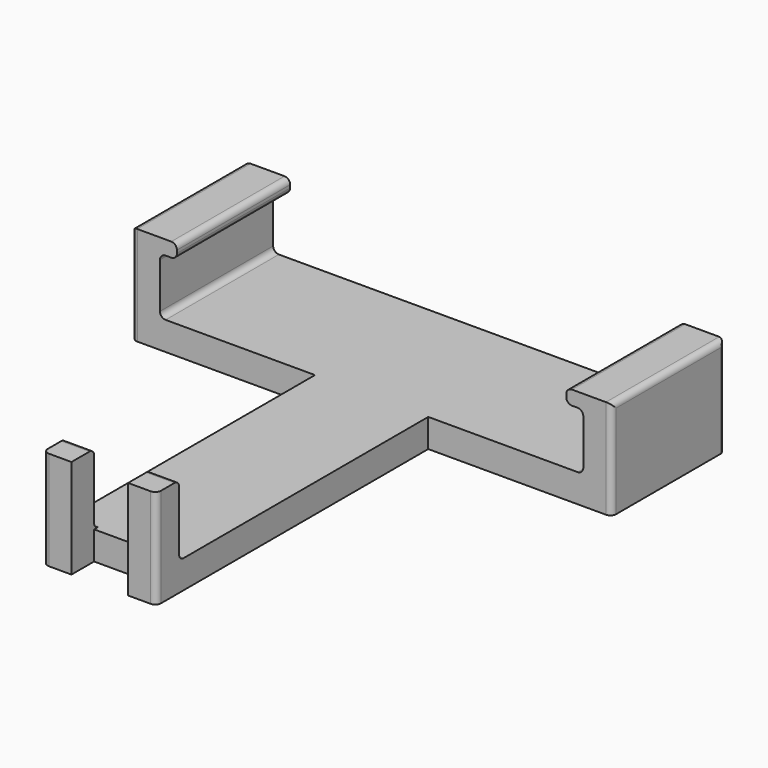
from build123d import *

# Parameters (mm, degrees)
F0_W     = 27.375
F0_H     = 25
F0_W_2   = 20
F0_H_2   = 55
F1_DEPTH = 5
F2_W     = 5
F2_H     = 25
F2_H_2   = 5
F3_DEPTH = 17.5
F4_W     = 25
F4_H     = 2.5
F5_DEPTH = 3
F6_W     = 25
F6_H     = 2.5
F7_DEPTH = 3
F8_R     = 1


with BuildPart() as f1:
    # F0 (on Top) → F1 (new body)
    with BuildSketch(Plane.XY):
        with Locations((-23.6875, 0)):
            Rectangle(F0_W, F0_H)
        Rectangle(F0_W_2, F0_H)
        with Locations((23.6875, 0)):
            Rectangle(F0_W, F0_H)
        with Locations((0, -40)):
            Rectangle(F0_W_2, F0_H_2)
    extrude(amount=F1_DEPTH)

    # F2 (on Top) → F3 (join)
    with BuildSketch(Plane.XY):
        with Locations((-39.875, 0)):
            Rectangle(F2_W, F2_H)
        with Locations((39.875, 0)):
            Rectangle(F2_W, F2_H)
        with Locations((-7.5, -70)):
            Rectangle(F2_W, F2_H_2)
        with Locations((7.5, -70)):
            Rectangle(F2_W, F2_H_2)
    extrude(amount=F3_DEPTH)

    # F4 (on face) → F5 (join)
    with BuildSketch(Plane.YZ.offset(-37.375)):
        with Locations((0, 16.25)):
            Rectangle(F4_W, F4_H)
    extrude(amount=F5_DEPTH)

    # F6 (on face) → F7 (join)
    with BuildSketch(Plane(origin=(37.375, 0, 0), x_dir=(0, -1, 0), z_dir=(-1, 0, 0))):
        with Locations((0, 16.25)):
            Rectangle(F6_W, F6_H)
    extrude(amount=F7_DEPTH)

    # F8
    f8_edges = [f1.edges().sort_by_distance(p)[0] for p in [
        (-37.375, 0, 5),
        (37.375, 0, 5),
        (7.5, -67.5, 17.5),
        (-7.5, -67.5, 17.5),
        (7.5, -67.5, 5),
        (-7.5, -67.5, 5),
        (-42.375, -12.5, 8.75),
        (-42.375, 12.5, 8.75),
        (-42.375, 0, 17.5),
        (42.375, 0, 17.5),
        (42.375, -12.5, 8.75),
        (42.375, 12.5, 8.75),
        (-10, -72.5, 8.75),
        (10, -72.5, 8.75),
        (-34.375, 0, 17.5),
        (-34.375, 0, 15),
        (34.375, 0, 17.5),
        (34.375, 0, 15),
        (37.375, 0, 15),
        (-37.375, 0, 15),
    ]]
    fillet(f8_edges, radius=F8_R)


solid = f1.part
